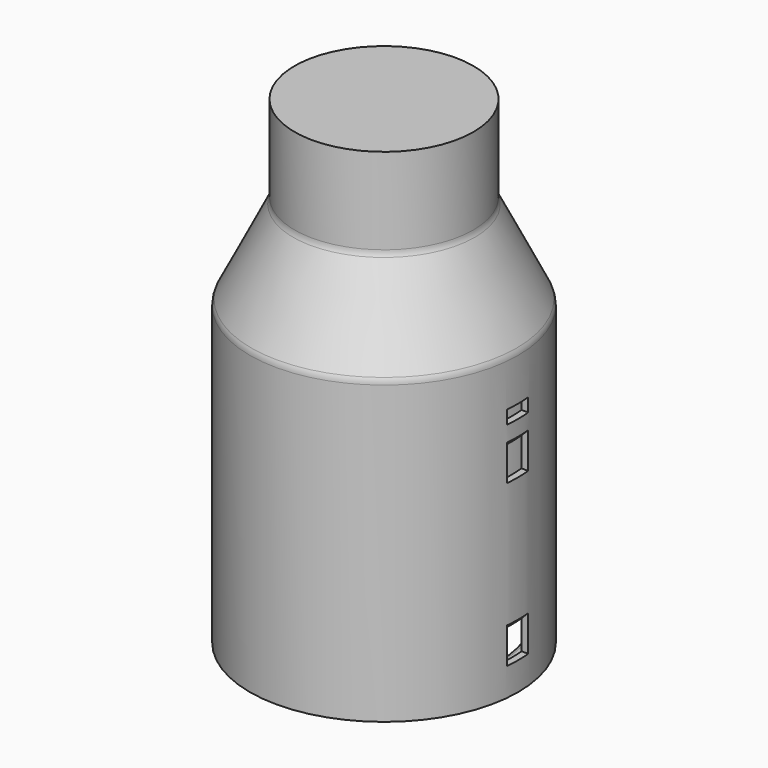
from build123d import *

# Parameters (mm, degrees)
F2_W         = 5.9824174088
F2_H         = 6
F2_H_2       = 3
F3_DEPTH     = 25
F4_T4_ANGLE  = 15.5454173813
F4_T9_ANGLE  = 15.5454173813
F4_T14_ANGLE = 15.5454173813
F4_T19_ANGLE = 15.5454173813


# Not quite as in the source:
# - a fillet or chamfer that OpenCascade refuses, or shapes differently, is made with other operations: its cross-section is extruded or revolved along the edge and cut away or added


with BuildPart() as f1:
    # F0 (on Front) → F1 (revolve)
    with BuildSketch(Plane.XZ):
        with BuildLine():
            Line((-1.8438853237, 0), (0, 0))
            Line((0, 0), (0, 66.2917960675))
            ThreePointArc((0, 66.2917960675), (-0.0802530316, 66.9810548291), (-0.316718427, 67.633436854))
            Line((-0.316718427, 67.633436854), (-9.683281573, 86.366563146))
            ThreePointArc((-9.683281573, 86.366563146), (-9.9197469684, 87.0189451709), (-10, 87.7082039325))
            Line((-10, 87.7082039325), (-10, 107))
            Line((-10, 107), (-30, 107))
            Line((-30, 107), (-30, 105.5))
            Line((-30, 105.5), (-26.5, 105.5))
            ThreePointArc((-26.5, 105.5), (-15.8933982822, 101.1066017178), (-11.5, 90.5))
            Line((-11.5, 90.5), (-11.5, 87.7082039325))
            ThreePointArc((-11.5, 87.7082039325), (-11.3796204526, 86.67431579), (-11.0249223595, 85.6957427527))
            Line((-11.0249223595, 85.6957427527), (-2.027864045, 67.7016261238))
            ThreePointArc((-2.027864045, 67.7016261238), (-1.6337550527, 66.614322749), (-1.5, 65.4655581463))
            Line((-1.5, 65.4655581463), (-1.5, 6))
            ThreePointArc((-1.5, 6), (-1.7928932188, 5.2928932188), (-2.5, 5))
            Line((-2.5, 5), (-3.5, 5))
            ThreePointArc((-3.5, 5), (-4.2071067812, 4.7071067812), (-4.5, 4))
            ThreePointArc((-4.5, 4), (-4.2071067812, 3.2928932188), (-3.5, 3))
            Line((-3.5, 3), (-3, 3))
            ThreePointArc((-3, 3), (-2.2928932188, 2.7071067812), (-2, 2))
            Line((-2, 2), (-2, 0.1561146763))
            ThreePointArc((-2, 0.1561146763), (-1.9542750699, 0.0457249301), (-1.8438853237, 0))
        make_face()
    revolve(axis=Axis((-30, 0, 106.25), (0, 0, -1)))

    # F2 (on Right) → F3 (cut)
    with BuildSketch(Plane.YZ):
        with Locations((0, 9.2917960675)):
            Rectangle(F2_W, F2_H)
        with Locations((0, 45.2917960675)):
            Rectangle(F2_W, F2_H)
        with Locations((0, 55.2917960675)):
            Rectangle(F2_W, F2_H_2)
    extrude(amount=-F3_DEPTH, mode=Mode.SUBTRACT)

    # F4: chamfer of 2 on 4 edges, made by hand


with BuildPart() as f4_tool2:
    # F4_s3 → F4_t4 (revolve)
    with BuildSketch(Plane(origin=(-2.1547544976, -7.7459452608, 0), x_dir=(0, 0, 1), z_dir=(-0.2680021454, -0.9634183152, 0))):
        Polygon((50.2917960675, -1.0974505437), (48.2917960675, 0.9025494563), (48.2917960675, -1.0974505437), align=None)
    revolve(axis=Axis((-30, 0, 48.2917960675), (0, 0, 1)), revolution_arc=F4_T4_ANGLE)

    split(bisect_by=Plane.XZ.offset(2.9912087044), keep=Keep.BOTTOM)


with BuildPart() as f1_1:
    add(f1.part)

    # F4_t1: cut F4_tool2
    add(f4_tool2.part, mode=Mode.SUBTRACT)


with BuildPart() as f4_tool7:
    # F4_s8 → F4_t9 (revolve)
    with BuildSketch(Plane.XZ):
        Polygon((0, 50.2917960675), (-2, 48.2917960675), (0, 48.2917960675), align=None)
    revolve(axis=Axis((-30, 0, 48.2917960675), (0, 0, 1)), revolution_arc=F4_T9_ANGLE)

    split(bisect_by=Plane.XZ.offset(-2.9912087044), keep=Keep.TOP)


with BuildPart() as f1_2:
    add(f1_1.part)

    # F4_t6: cut F4_tool7
    add(f4_tool7.part, mode=Mode.SUBTRACT)


with BuildPart() as f4_tool12:
    # F4_s13 → F4_t14 (revolve)
    with BuildSketch(Plane(origin=(-2.1547544976, -7.7459452608, 0), x_dir=(0, 0, 1), z_dir=(-0.2680021454, -0.9634183152, 0))):
        Polygon((14.2917960675, -1.0974505437), (12.2917960675, 0.9025494563), (12.2917960675, -1.0974505437), align=None)
    revolve(axis=Axis((-30, 0, 12.2917960675), (0, 0, 1)), revolution_arc=F4_T14_ANGLE)

    split(bisect_by=Plane.XZ.offset(2.9912087044), keep=Keep.BOTTOM)


with BuildPart() as f1_3:
    add(f1_2.part)

    # F4_t11: cut F4_tool12
    add(f4_tool12.part, mode=Mode.SUBTRACT)


with BuildPart() as f4_tool17:
    # F4_s18 → F4_t19 (revolve)
    with BuildSketch(Plane.XZ):
        Polygon((0, 14.2917960675), (-2, 12.2917960675), (0, 12.2917960675), align=None)
    revolve(axis=Axis((-30, 0, 12.2917960675), (0, 0, 1)), revolution_arc=F4_T19_ANGLE)

    split(bisect_by=Plane.XZ.offset(-2.9912087044), keep=Keep.TOP)


with BuildPart() as f1_4:
    add(f1_3.part)

    # F4_t16: cut F4_tool17
    add(f4_tool17.part, mode=Mode.SUBTRACT)


solid = f1_4.part
